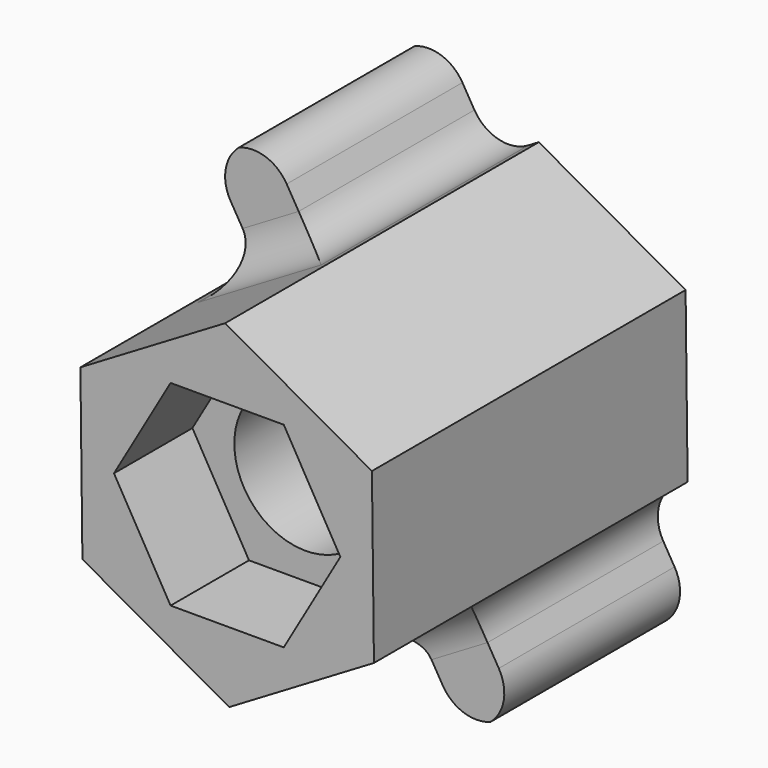
from build123d import *

# Parameters (mm, degrees)
F1_DEPTH      = 20
F2_DEPTH      = 15
F4_W          = 3.3256819006
F4_H          = 11.2064601853
F5_DEPTH      = 5.2
F5_DEPTH_BACK = 20
F3_R          = 3.6353661433
F6_DEPTH      = 25
F7_T1_DEPTH   = 11.2064601853
F7_T3_DEPTH   = 3.3256819006
F7_T5_DEPTH   = 3.3256819006
F7_T11_DEPTH  = 8.3256819006
F7_T16_DEPTH  = 16.2064601853
F7_T23_DEPTH  = 16.2064601853
F7_T27_DEPTH  = 8.3256819006
F7_T35_DEPTH  = 8.3256819006
F7_T40_DEPTH  = 16.2064601853
F7_T47_DEPTH  = 16.2064601853
F7_T51_DEPTH  = 8.3256819006
F7_T55_DEPTH  = 21.2064601853


# Not quite as in the source:
# - a fillet or chamfer that OpenCascade refuses, or shapes differently, is made with other operations: its cross-section is extruded or revolved along the edge and cut away or added


with BuildPart() as f1:
    # F0 (on Front) → F1 (new body)
    with BuildSketch(Plane.XZ):
        Polygon((7.3840099636, 4.3827313822), (-0.1035517331, 8.5861059014), (-7.4875616967, 4.2033745192), (-7.3840099636, -4.3827313822), (0.1035517331, -8.5861059014), (7.4875616967, -4.2033745192), align=None)
        Polygon((-2.8867513459, 5), (2.8867513459, 5), (5.7735026919, 0), (2.8867513459, -5), (-2.8867513459, -5), (-5.7735026919, 0), align=None, mode=Mode.SUBTRACT)
    extrude(amount=F1_DEPTH)

    # F0 (on Front) → F2 (join)
    with BuildSketch(Plane.XZ):
        Polygon((5.7735026919, 0), (2.8867513459, 5), (-2.8867513459, 5), (-5.7735026919, 0), (-2.8867513459, -5), (2.8867513459, -5), align=None)
    extrude(amount=F2_DEPTH)

    # F4 (on face) → F5 (join, two sides)
    with BuildSketch(Plane(origin=(-3.7955567149, 0, 6.3947402103), x_dir=(0.8599326743, 0, 0.51040748), z_dir=(-0.51040748, 0, 0.8599326743))) as f5_sk:
        with Locations((0, -5.6032300927)):
            Rectangle(F4_W, F4_H)
    extrude(amount=F5_DEPTH)
    extrude(f5_sk.sketch, amount=-F5_DEPTH_BACK)

    # F3 (on face) → F6 (cut)
    with BuildSketch(Plane.XZ.offset(15)):
        Circle(F3_R)
    extrude(amount=-F6_DEPTH, mode=Mode.SUBTRACT)

    # F7: fillet of radius 2 on 10 edges, made by hand

    # F7_s2 → F7_t1 (join)
    with BuildSketch(Plane.XZ):
        with BuildLine():
            ThreePointArc((-6.9453533288, 4.525198791), (-6.0282146576, 5.7507608695), (-6.2463029403, 7.2658790997))
            Line((-6.2463029403, 7.2658790997), (-5.2254879802, 5.5460137511))
            Line((-5.2254879802, 5.5460137511), (-6.9453533288, 4.525198791))
        make_face()
        with BuildLine():
            ThreePointArc((-0.645760101, 8.2642816296), (-2.1608783312, 8.0461933468), (-3.3864404097, 8.963332018))
            Line((-3.3864404097, 8.963332018), (-2.3656254496, 7.2434666695))
            Line((-2.3656254496, 7.2434666695), (-0.645760101, 8.2642816296))
        make_face()
        with BuildLine():
            ThreePointArc((6.9453533288, -4.525198791), (6.0282146576, -5.7507608695), (6.2463029403, -7.2658790997))
            Line((6.2463029403, -7.2658790997), (5.2254879802, -5.5460137511))
            Line((5.2254879802, -5.5460137511), (6.9453533288, -4.525198791))
        make_face()
        with BuildLine():
            ThreePointArc((0.645760101, -8.2642816296), (2.1608783312, -8.0461933468), (3.3864404097, -8.963332018))
            Line((3.3864404097, -8.963332018), (2.3656254496, -7.2434666695))
            Line((2.3656254496, -7.2434666695), (0.645760101, -8.2642816296))
        make_face()
    extrude(amount=F7_T1_DEPTH)

    # F7_s4 → F7_t3 (join)
    with BuildSketch(Plane(origin=(-1.4299312653, 0, -0.8487264592), x_dir=(0, 1, 0), z_dir=(0.8599326743, 0, 0.51040748))):
        with BuildLine():
            ThreePointArc((-13.2064601853, 7.4363265887), (-11.792246623, 8.0221130263), (-11.2064601853, 9.4363265887))
            Line((-11.2064601853, 9.4363265887), (-11.2064601853, 7.4363265887))
            Line((-11.2064601853, 7.4363265887), (-13.2064601853, 7.4363265887))
        make_face()
    extrude(amount=F7_T3_DEPTH)

    # F7_s6 → F7_t5 (join)
    with BuildSketch(Plane(origin=(1.4299312653, 0, 0.8487264592), x_dir=(0, 1, 0), z_dir=(-0.8599326743, 0, -0.51040748))):
        with BuildLine():
            ThreePointArc((-13.2064601853, 7.4363265887), (-11.792246623, 8.0221130263), (-11.2064601853, 9.4363265887))
            Line((-11.2064601853, 9.4363265887), (-11.2064601853, 7.4363265887))
            Line((-11.2064601853, 7.4363265887), (-13.2064601853, 7.4363265887))
        make_face()
    extrude(amount=F7_T5_DEPTH)


with BuildPart() as f7_tool9:
    # F7_s10 → F7_t11 (new body)
    with BuildSketch(Plane(origin=(-5.7295946368, 0, -3.4007638594), x_dir=(0, 1, 0), z_dir=(0.8599326743, 0, 0.51040748))):
        with BuildLine():
            ThreePointArc((-13.2064601853, 7.4363265887), (-11.792246623, 8.0221130263), (-11.2064601853, 9.4363265887))
            Line((-11.2064601853, 9.4363265887), (-11.2064601853, 7.4363265887))
            Line((-11.2064601853, 7.4363265887), (-13.2064601853, 7.4363265887))
        make_face()
    extrude(amount=F7_T11_DEPTH)

    split(bisect_by=Plane(origin=(-7.4357858302, 0, -0.0896784315), x_dir=(0, 1, 0), z_dir=(0.9999272815, 0, 0.0120595069)), keep=Keep.TOP)

    split(bisect_by=Plane(origin=(-1.4299312653, 0, -0.8487264592), x_dir=(0, 1, 0), z_dir=(-0.8599326743, 0, -0.51040748)), keep=Keep.TOP)


with BuildPart() as f7_tool14:
    # F7_s15 → F7_t16 (new body)
    with BuildSketch(Plane.XZ):
        with BuildLine():
            ThreePointArc((-6.9453533288, 4.525198791), (-6.0282146576, 5.7507608695), (-6.2463029403, 7.2658790997))
            Line((-6.2463029403, 7.2658790997), (-5.2254879802, 5.5460137511))
            Line((-5.2254879802, 5.5460137511), (-6.9453533288, 4.525198791))
        make_face()
    extrude(amount=F7_T16_DEPTH)

    split(bisect_by=Plane.XZ.offset(11.2064601853), keep=Keep.TOP)


with BuildPart() as f7_tool9_1:
    add(f7_tool9.part)

    # F7_t18: intersect F7_tool14
    add(f7_tool14.part, mode=Mode.INTERSECT)


with BuildPart() as f1_1:
    add(f1.part)

    # F7_t7: union F7_tool9
    add(f7_tool9_1.part)


with BuildPart() as f7_tool21:
    # F7_s22 → F7_t23 (new body)
    with BuildSketch(Plane.XZ.offset(16.2064601853)):
        with BuildLine():
            ThreePointArc((-0.645760101, 8.2642816296), (-2.1608783312, 8.0461933468), (-3.3864404097, 8.963332018))
            Line((-3.3864404097, 8.963332018), (-2.3656254496, 7.2434666695))
            Line((-2.3656254496, 7.2434666695), (-0.645760101, 8.2642816296))
        make_face()
    extrude(amount=-F7_T23_DEPTH)

    split(bisect_by=Plane.XZ.offset(11.2064601853), keep=Keep.TOP)


with BuildPart() as f7_tool25:
    # F7_s26 → F7_t27 (new body)
    with BuildSketch(Plane(origin=(-1.4299312653, 0, -0.8487264592), x_dir=(0, 1, 0), z_dir=(0.8599326743, 0, 0.51040748))):
        with BuildLine():
            ThreePointArc((-13.2064601853, 7.4363265887), (-11.792246623, 8.0221130263), (-11.2064601853, 9.4363265887))
            Line((-11.2064601853, 9.4363265887), (-11.2064601853, 7.4363265887))
            Line((-11.2064601853, 7.4363265887), (-13.2064601853, 7.4363265887))
        make_face()
    extrude(amount=F7_T27_DEPTH)

    split(bisect_by=Plane(origin=(3.6402291153, 0, 6.4844186418), x_dir=(0, 1, 0), z_dir=(-0.4895198015, 0, -0.8719921811)), keep=Keep.TOP)

    split(bisect_by=Plane(origin=(1.4299312653, 0, 0.8487264592), x_dir=(0, 1, 0), z_dir=(0.8599326743, 0, 0.51040748)), keep=Keep.TOP)


with BuildPart() as f7_tool21_1:
    add(f7_tool21.part)

    # F7_t30: intersect F7_tool25
    add(f7_tool25.part, mode=Mode.INTERSECT)


with BuildPart() as f1_2:
    add(f1_1.part)

    # F7_t19: union F7_tool21
    add(f7_tool21_1.part)


with BuildPart() as f7_tool33:
    # F7_s34 → F7_t35 (new body)
    with BuildSketch(Plane(origin=(5.7295946368, 0, 3.4007638594), x_dir=(0, 1, 0), z_dir=(-0.8599326743, 0, -0.51040748))):
        with BuildLine():
            ThreePointArc((-13.2064601853, 7.4363265887), (-11.792246623, 8.0221130263), (-11.2064601853, 9.4363265887))
            Line((-11.2064601853, 9.4363265887), (-11.2064601853, 7.4363265887))
            Line((-11.2064601853, 7.4363265887), (-13.2064601853, 7.4363265887))
        make_face()
    extrude(amount=F7_T35_DEPTH)

    split(bisect_by=Plane(origin=(7.4357858302, 0, 0.0896784315), x_dir=(0, 1, 0), z_dir=(-0.9999272815, 0, -0.0120595069)), keep=Keep.TOP)

    split(bisect_by=Plane(origin=(1.4299312653, 0, 0.8487264592), x_dir=(0, 1, 0), z_dir=(0.8599326743, 0, 0.51040748)), keep=Keep.TOP)


with BuildPart() as f7_tool38:
    # F7_s39 → F7_t40 (new body)
    with BuildSketch(Plane.XZ):
        with BuildLine():
            ThreePointArc((6.9453533288, -4.525198791), (6.0282146576, -5.7507608695), (6.2463029403, -7.2658790997))
            Line((6.2463029403, -7.2658790997), (5.2254879802, -5.5460137511))
            Line((5.2254879802, -5.5460137511), (6.9453533288, -4.525198791))
        make_face()
    extrude(amount=F7_T40_DEPTH)

    split(bisect_by=Plane.XZ.offset(11.2064601853), keep=Keep.TOP)


with BuildPart() as f7_tool33_1:
    add(f7_tool33.part)

    # F7_t42: intersect F7_tool38
    add(f7_tool38.part, mode=Mode.INTERSECT)


with BuildPart() as f1_3:
    add(f1_2.part)

    # F7_t31: union F7_tool33
    add(f7_tool33_1.part)


with BuildPart() as f7_tool45:
    # F7_s46 → F7_t47 (new body)
    with BuildSketch(Plane.XZ.offset(16.2064601853)):
        with BuildLine():
            ThreePointArc((0.645760101, -8.2642816296), (2.1608783312, -8.0461933468), (3.3864404097, -8.963332018))
            Line((3.3864404097, -8.963332018), (2.3656254496, -7.2434666695))
            Line((2.3656254496, -7.2434666695), (0.645760101, -8.2642816296))
        make_face()
    extrude(amount=-F7_T47_DEPTH)

    split(bisect_by=Plane.XZ.offset(11.2064601853), keep=Keep.TOP)


with BuildPart() as f7_tool49:
    # F7_s50 → F7_t51 (new body)
    with BuildSketch(Plane(origin=(1.4299312653, 0, 0.8487264592), x_dir=(0, 1, 0), z_dir=(-0.8599326743, 0, -0.51040748))):
        with BuildLine():
            ThreePointArc((-13.2064601853, 7.4363265887), (-11.792246623, 8.0221130263), (-11.2064601853, 9.4363265887))
            Line((-11.2064601853, 9.4363265887), (-11.2064601853, 7.4363265887))
            Line((-11.2064601853, 7.4363265887), (-13.2064601853, 7.4363265887))
        make_face()
    extrude(amount=F7_T51_DEPTH)

    split(bisect_by=Plane(origin=(-3.6402291153, 0, -6.4844186418), x_dir=(0, 1, 0), z_dir=(0.4895198015, 0, 0.8719921811)), keep=Keep.TOP)

    split(bisect_by=Plane(origin=(-1.4299312653, 0, -0.8487264592), x_dir=(0, 1, 0), z_dir=(-0.8599326743, 0, -0.51040748)), keep=Keep.TOP)


with BuildPart() as f7_tool45_1:
    add(f7_tool45.part)

    # F7_t54: intersect F7_tool49
    add(f7_tool49.part, mode=Mode.INTERSECT)


with BuildPart() as f1_4:
    add(f1_3.part)

    # F7_t43: union F7_tool45
    add(f7_tool45_1.part)

    # F7_s56 → F7_t55 (cut)
    with BuildSketch(Plane.XZ.offset(-5)):
        with BuildLine():
            ThreePointArc((-6.1597415279, 11.0384786175), (-7.0768801991, 9.8129165391), (-6.8587919164, 8.2977983089))
            Line((-6.8587919164, 8.2977983089), (-7.8796068765, 10.0176636575))
            Line((-7.8796068765, 10.0176636575), (-6.1597415279, 11.0384786175))
        make_face()
        with BuildLine():
            ThreePointArc((-3.9989293858, 9.9952512272), (-5.2244914642, 10.9123898984), (-6.7396096944, 10.6943016157))
            Line((-6.7396096944, 10.6943016157), (-5.0197443458, 11.7151165758))
            Line((-5.0197443458, 11.7151165758), (-3.9989293858, 9.9952512272))
        make_face()
        with BuildLine():
            ThreePointArc((6.7025269693, -10.6318247746), (5.1874087391, -10.8499130573), (3.9618466606, -9.9327743861))
            Line((3.9618466606, -9.9327743861), (4.9826616207, -11.6526397347))
            Line((4.9826616207, -11.6526397347), (6.7025269693, -10.6318247746))
        make_face()
        with BuildLine():
            ThreePointArc((6.8217091912, -8.2353214678), (7.039797474, -9.750439698), (6.1226588027, -10.9760017765))
            Line((6.1226588027, -10.9760017765), (7.8425241513, -9.9551868164))
            Line((7.8425241513, -9.9551868164), (6.8217091912, -8.2353214678))
        make_face()
    extrude(amount=F7_T55_DEPTH, mode=Mode.SUBTRACT)


solid = f1_4.part
